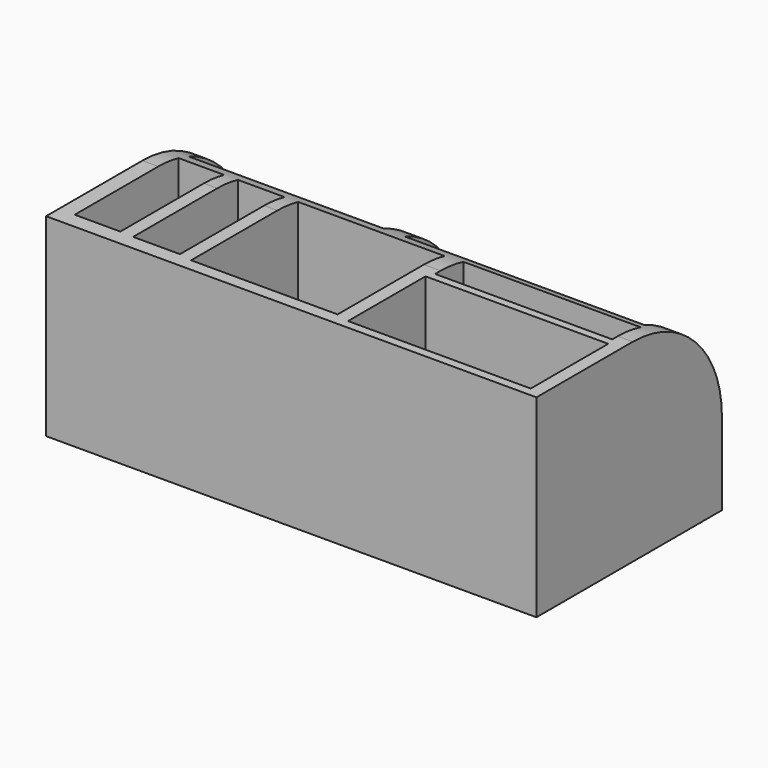
from build123d import *

# Parameters (mm, degrees)
F0_W         = 198.7862437963
F0_H         = 84.2363908887
F1_DEPTH     = 87.63
F2_DEPTH     = 30.226
F3_DEPTH     = 38.1
F4_DEPTH     = 36.068
F5_W         = 118.6288297176
F5_H         = 62.8803037107
F6_DEPTH     = 119.38
F7_W         = 114.9956956506
F7_H         = 23.0015479028
F8_DEPTH     = 114.3
F9_DEPTH     = 216.916
F10_DEPTH    = 97.282
F11_W        = 95.1088294387
F11_H        = 86.9466327131
F14_DEPTH    = 121.666
F12_W        = 30.4002016783
F12_H        = 84.9931621924
F15_DEPTH    = 121.666
F13_W        = 29.6071916819
F13_H        = 84.3174913898
F16_DEPTH    = 121.666
F18_W        = 155.8008268476
F18_H        = 43.2829973288
F19_DEPTH    = 121.666
F17_W        = 126.6549825668
F17_H        = 42.8492124192
F20_DEPTH    = 121.666
F21_T1_DEPTH = 680.2142882536


# Not quite as in the source:
# - a fillet or chamfer that OpenCascade refuses, or shapes differently, is made with other operations: its cross-section is extruded or revolved along the edge and cut away or added


with BuildPart() as f1:
    # F0 (on Top) → F1 (new body)
    with BuildSketch(Plane.XY):
        Rectangle(F0_W, F0_H)
    extrude(amount=F1_DEPTH)

    # F2 (add): a face of the model
    f2_faces = [f1.faces().sort_by_distance(p)[0] for p in [
        (0, -42.1181954443, 43.815),
    ]]
    extrude(f2_faces, amount=F2_DEPTH)

    # F3 (add): a face of the model
    f3_faces = [f1.faces().sort_by_distance(p)[0] for p in [
        (0, -15.113, 0),
    ]]
    extrude(f3_faces, amount=F3_DEPTH)

    # F4 (add): a face of the model
    f4_faces = [f1.faces().sort_by_distance(p)[0] for p in [
        (0, -72.3441954443, 24.765),
    ]]
    extrude(f4_faces, amount=F4_DEPTH)

    # F5 (on face) → F6 (cut)
    with BuildSketch(Plane.XY.offset(87.63)):
        with Locations((31.7698940635, -71.2347794324)):
            Rectangle(F5_W, F5_H)
    extrude(amount=-F6_DEPTH, mode=Mode.SUBTRACT)

    # F7 (on face) → F8 (cut)
    with BuildSketch(Plane.XY.offset(87.63)):
        with Locations((32.1380235255, -23.2001785189)):
            Rectangle(F7_W, F7_H)
    extrude(amount=-F8_DEPTH, mode=Mode.SUBTRACT)

    # F9 (add): a face of the model
    f9_faces = [f1.faces().sort_by_distance(p)[0] for p in [
        (-99.3931218982, -33.147, 24.765),
    ]]
    extrude(f9_faces, amount=F9_DEPTH)

    # F10 (cut): a face of the model
    f10_faces = [f1.faces().sort_by_distance(p)[0] for p in [
        (-316.3091218982, -33.147, 24.765),
    ]]
    extrude(f10_faces, amount=-F10_DEPTH, mode=Mode.SUBTRACT)

    # F11 (on face) → F14 (cut)
    with BuildSketch(Plane.XY.offset(87.63)):
        with Locations((-83.8001854718, -56.8147618324)):
            Rectangle(F11_W, F11_H)
    extrude(amount=-F14_DEPTH, mode=Mode.SUBTRACT)

    # F12 (on face) → F15 (cut)
    with BuildSketch(Plane.XY.offset(87.63)):
        with Locations((-155.1787778735, -56.0720595531)):
            Rectangle(F12_W, F12_H)
    extrude(amount=-F15_DEPTH, mode=Mode.SUBTRACT)

    # F13 (on face) → F16 (cut)
    with BuildSketch(Plane.XY.offset(87.63)):
        with Locations((-193.8888058066, -55.9172849171)):
            Rectangle(F13_W, F13_H)
    extrude(amount=-F16_DEPTH, mode=Mode.SUBTRACT)

    # F18 (on face) → F19 (cut)
    with BuildSketch(Plane.XY.offset(87.63)):
        with Locations((9.4717927277, 15.8045829739)):
            Rectangle(F18_W, F18_H)
    extrude(amount=-F19_DEPTH, mode=Mode.SUBTRACT)

    # F17 (on face) → F20 (cut)
    with BuildSketch(Plane.XY.offset(87.63)):
        with Locations((-145.3649103642, 15.8879833762)):
            Rectangle(F17_W, F17_H)
    extrude(amount=-F20_DEPTH, mode=Mode.SUBTRACT)

    # F21: fillet of radius 72.3588088914 on 1 edges, made by hand

    # F21_s2 → F21_t1 (cut)
    with BuildSketch(Plane.YZ.offset(-399.9241441268)):
        with BuildLine():
            ThreePointArc((42.1181954443, 15.2711911086), (20.9247909986, 66.4365955543), (-30.2406134471, 87.63))
            Line((-30.2406134471, 87.63), (42.1181954443, 87.63))
            Line((42.1181954443, 87.63), (42.1181954443, 15.2711911086))
        make_face()
    extrude(amount=F21_T1_DEPTH, mode=Mode.SUBTRACT)


solid = f1.part
